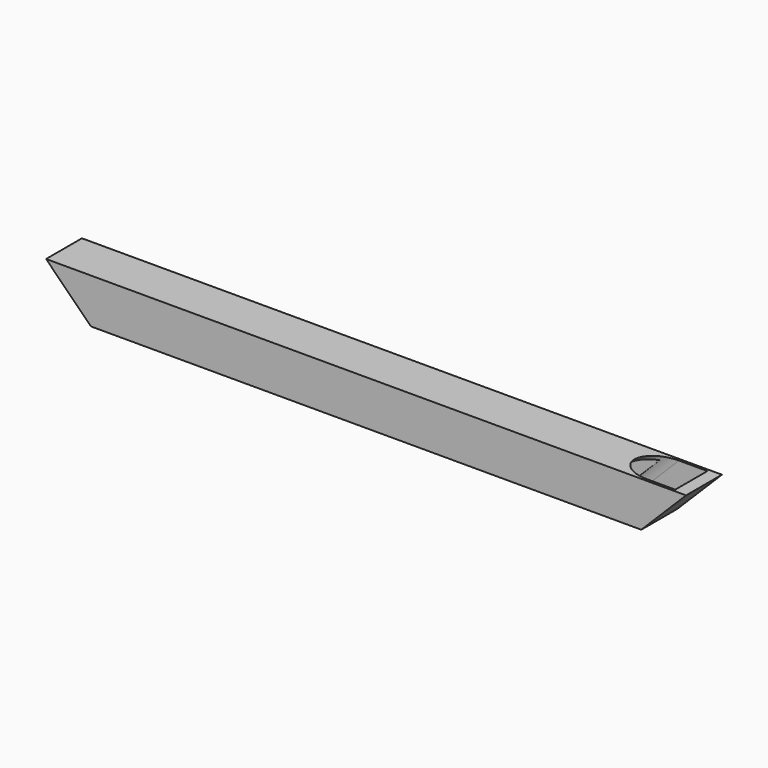
from build123d import *

# Parameters (mm, degrees)
F0_W         = 30
F0_H         = 30
F0_W_2       = 24
F0_H_2       = 24
F1_DEPTH     = 100
F3_DEPTH     = 30
F5_DEPTH     = 30
F7_DEPTH     = 6
F9_DEPTH     = 50
F13_W        = 30
F13_H        = 30
F14_DEPTH    = 30
F12_W        = 30
F12_H        = 30
F12_W_2      = 23.9601944461
F12_H_2      = 23.7035881728
F15_DEPTH    = 350
F16_T1_DEPTH = 184.300979278
F18_DEPTH    = 44.18
F19_SIZE     = 5.99
F20_SIZE     = 5.99999


# Not quite as in the source:
# - a fillet or chamfer that OpenCascade refuses, or shapes differently, is made with other operations: its cross-section is extruded or revolved along the edge and cut away or added
# - a fillet or chamfer is up to 0.001 mm smaller than in the source, because OpenCascade refuses the exact size


with BuildPart() as f1:
    # F0 (on Right) → F1 (new body)
    with BuildSketch(Plane.YZ):
        Rectangle(F0_W, F0_H)
        Rectangle(F0_W_2, F0_H_2, mode=Mode.SUBTRACT)
    extrude(amount=F1_DEPTH)

    # F2 (on face) → F3 (cut)
    with BuildSketch(Plane(origin=(0, 15, 0), x_dir=(-1, 0, 0), z_dir=(0, 1, 0))):
        Polygon((0, 15), (-30, -15), (0, -15), align=None)
    extrude(amount=-F3_DEPTH, mode=Mode.SUBTRACT)

    # F4 (on face) → F5 (cut)
    with BuildSketch(Plane.XZ.offset(15)):
        Polygon((70, -15), (100, -15), (100, 15), align=None)
    extrude(amount=-F5_DEPTH, mode=Mode.SUBTRACT)

    # F6 (on face) → F7 (join)
    with BuildSketch(Plane(origin=(42.5, 0, -42.5), x_dir=(0, 1, 0), z_dir=(0.7071067812, 0, -0.7071067812))):
        Polygon((-15, 38.8908729653), (15, 38.8908729653), (15, 43.1335136524), (12, 43.1335136524), (-12, 43.1335136524), (-15, 43.1335136524), align=None)
    extrude(amount=F7_DEPTH)

    # F8 (on face) → F9 (cut, symmetric)
    with BuildSketch(Plane(origin=(27.5, 0, 27.5), x_dir=(0, -1, 0), z_dir=(-0.7071067812, 0, -0.7071067812))):
        with BuildLine():
            ThreePointArc((9.63e-08, -60.1040764009), (9.510586241, -56.1646625738), (13.45, -46.6540764009))
            ThreePointArc((13.45, -46.6540764009), (0, -33.2040764009), (-13.45, -46.6540764009))
            ThreePointArc((-13.45, -46.6540764009), (-9.5105861729, -56.1646626419), (9.63e-08, -60.1040764009))
        make_face()
        with BuildLine():
            Line((13.45, -60.1040764009), (13.45, -46.6540764009))
            ThreePointArc((13.45, -46.6540764009), (9.510586241, -56.1646625738), (9.63e-08, -60.1040764009))
            Line((9.63e-08, -60.1040764009), (13.45, -60.1040764009))
        make_face()
        with BuildLine():
            ThreePointArc((9.63e-08, -60.1040764009), (-9.5105861729, -56.1646626419), (-13.45, -46.6540764009))
            Line((-13.45, -46.6540764009), (-13.45, -60.1040764009))
            Line((-13.45, -60.1040764009), (9.63e-08, -60.1040764009))
        make_face()
    extrude(amount=F9_DEPTH, both=True, mode=Mode.SUBTRACT)

    # F13 (on face) → F14 (cut)
    with BuildSketch(Plane(origin=(0, 15, 0), x_dir=(-1, 0, 0), z_dir=(0, 1, 0))):
        with Locations((-15, 0)):
            Rectangle(F13_W, F13_H)
    extrude(amount=-F14_DEPTH, mode=Mode.SUBTRACT)

    # F12 (on face) → F15 (join)
    with BuildSketch(Plane.YZ.offset(30)):
        Rectangle(F12_W, F12_H)
        with Locations((0.0199027769, -0.1482059136)):
            Rectangle(F12_W_2, F12_H_2, mode=Mode.SUBTRACT)
    extrude(amount=-F15_DEPTH)

    # F16: chamfer of 30 on 1 edges, made by hand

    # F16_s2 → F16_t1 (cut)
    with BuildSketch(Plane.XZ.offset(-92.150489639)):
        Polygon((-290, -15), (-320, 15), (-320, -15), align=None)
    extrude(amount=F16_T1_DEPTH, mode=Mode.SUBTRACT)

    # F17 (on face) → F18 (join)
    with BuildSketch(Plane(origin=(30.5, 0, 30.5), x_dir=(0, 1, 0), z_dir=(0.7071067812, 0, 0.7071067812))):
        Polygon((-13.45, -60.1040764009), (-15, -60.1040764009), (-15, -66.1040764009), (15, -66.1040764009), (15, -60.1040764009), (13.45, -60.1040764009), align=None)
    extrude(amount=F18_DEPTH)

    # F19
    f19_edges = [f1.edges().sort_by_distance(p)[0] for p in [
        (104.239978, 0, 19.239978),
    ]]
    chamfer(f19_edges, length=F19_SIZE)

    # F20 (size 6 in the source; OpenCascade refuses exactly that, so slightly less here)
    f20_edges = [f1.edges().sort_by_distance(p)[0] for p in [
        (74.242641, 0, -19.242641),
    ]]
    chamfer(f20_edges, length=F20_SIZE)


solid = f1.part
